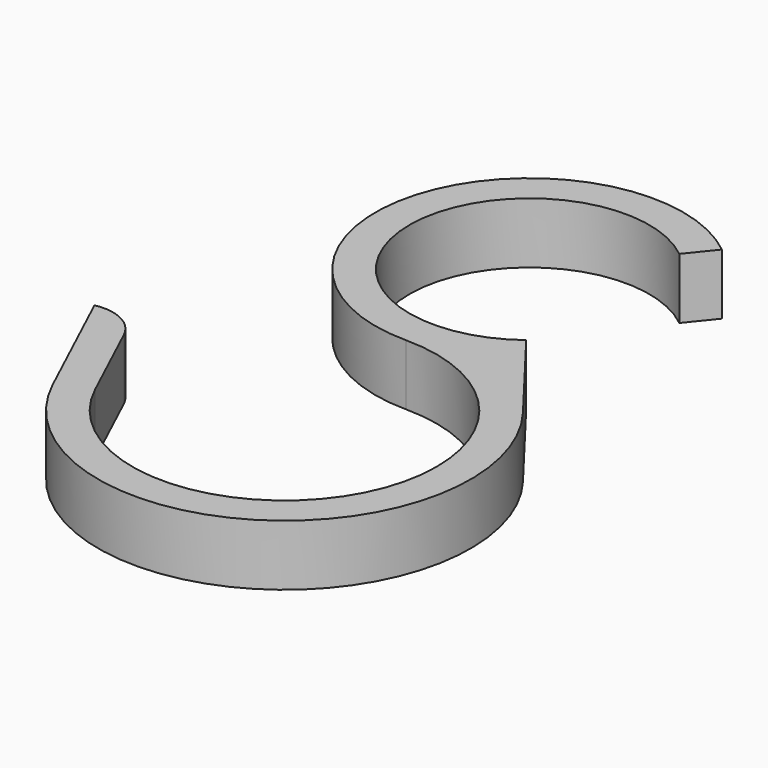
from build123d import *

# Parameters (mm, degrees)
F1_DEPTH    = 5
F2_T1_DEPTH = 22.6347624906


# Not quite as in the source:
# - a fillet or chamfer that OpenCascade refuses, or shapes differently, is made with other operations: its cross-section is extruded or revolved along the edge and cut away or added


with BuildPart() as f1:
    # F0 (on Top) → F1 (new body)
    with BuildSketch(Plane.XY):
        with BuildLine():
            ThreePointArc((5.9922465209, -7.8176391342), (-9.8492732487, 0.1196514659), (6.1803914025, 7.6697628458))
            Line((6.1803914025, 7.6697628458), (7.9372539332, 9.85))
            ThreePointArc((7.9372539332, 9.85), (-11.9294802904, 4.2083250825), (0, -12.65))
            ThreePointArc((0, -12.65), (8.8388347648, -16.3111652352), (12.5, -25.15))
            ThreePointArc((12.5, -25.15), (2.7054951742, -37.353700089), (-11.328847338, -30.4327282718))
            Line((-11.328847338, -30.4327282718), (-16.1166251075, -20.1653057112))
            Line((-16.1166251075, -20.1653057112), (-18.6542869112, -21.3486368441))
            Line((-18.6542869112, -21.3486368441), (-13.8665091417, -31.6160594046))
            ThreePointArc((-13.8665091417, -31.6160594046), (7.9338387883, -38.2322093731), (12.1431348989, -15.8422465209))
            Line((12.1431348989, -15.8422465209), (7.5500579161, -9.85))
            Line((7.5500579161, -9.85), (5.9922465209, -7.8176391342))
        make_face()
    extrude(amount=F1_DEPTH)

    # F2: fillet of radius 3.6213203436 on 1 edges, made by hand

    # F2_s2 → F2_t1 (cut)
    with BuildSketch(Plane.XY.offset(-8.8173812453)):
        with BuildLine():
            ThreePointArc((-14.6260705735, -23.3618102248), (-16.289199108, -21.6529383212), (-18.6542869112, -21.3486368441))
            Line((-18.6542869112, -21.3486368441), (-16.1166251075, -20.1653057112))
            Line((-16.1166251075, -20.1653057112), (-14.6260705735, -23.3618102248))
        make_face()
    extrude(amount=F2_T1_DEPTH, mode=Mode.SUBTRACT)


solid = f1.part
